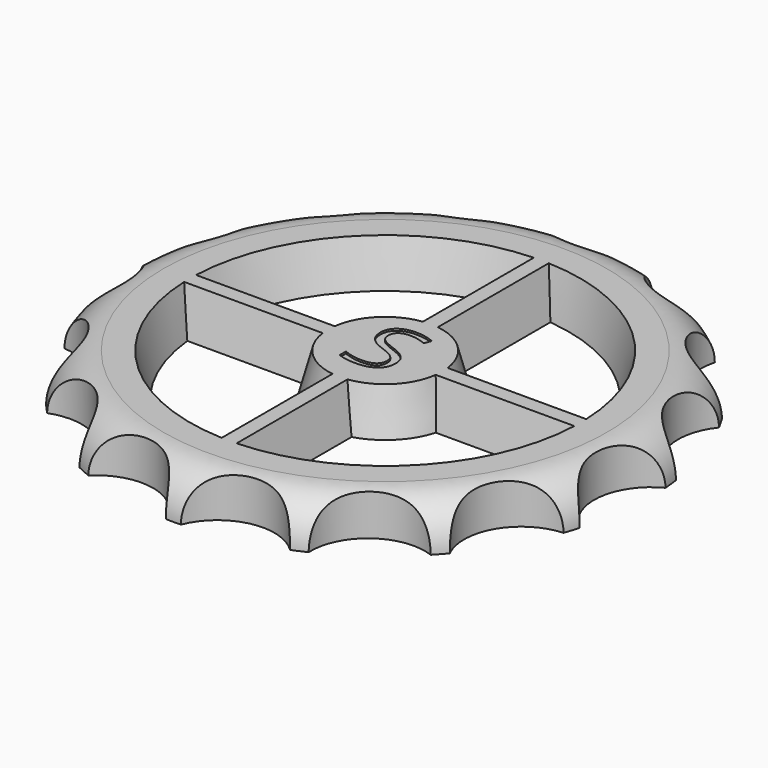
from build123d import *

# Parameters (mm, degrees)
F2_R                     = 15
F3_DEPTH                 = 25
F5_DEPTH                 = 25
DRAFT_F5_DRAFTED_ANGLE   = -15
DRAFT_F5_2_DRAFTED_ANGLE = -15
DRAFT_F5_3_DRAFTED_ANGLE = -15
DRAFT_F5_4_DRAFTED_ANGLE = -15
F6_TEXT_SIZE             = 25.1437097581
F7_DEPTH                 = 0.5


# Not quite as in the source:
# - an extrude with a draft is written as a straight extrude whose walls are then drafted
# - Text() gives the source's letters only with a copy of the font that has no kerning and outlines rounded to 1/6400 em; it was checked with that copy


with BuildPart() as f1:
    # F0 (on Front) → F1 (revolve)
    with BuildSketch(Plane.XZ):
        with BuildLine():
            Line((0, 11.3389009134), (-58.2126826048, 11.3389009134))
            ThreePointArc((-58.2126826048, 11.3389009134), (-66.2304963319, 8.0178137271), (-69.5515835182, 0))
            Line((-69.5515835182, 0), (0, 0))
            Line((0, 0), (0, 11.3389009134))
        make_face()
    revolve(axis=Axis((0, 0, 5.6694504567), (0, 0, 1)))

    # F2 (on Top) → F3 (cut)
    with BuildSketch(Plane.XY):
        with BuildLine():
            ThreePointArc((-0.9417421253, -75), (-12.820175043, -60.3284009409), (-29.6425179854, -68.8935492444))
            ThreePointArc((-29.6425179854, -68.8935492444), (-19.0633092075, -89.6715990591), (-0.9417421253, -75))
        make_face()
        with BuildLine():
            ThreePointArc((-30.0687543361, -62.0318186464), (-38.9650040167, -48.3298395179), (-55.1013186079, -50.8806907154))
            ThreePointArc((-55.1013186079, -50.8806907154), (-53.8855331205, -74.167073562), (-31.3631685962, -68.127466235))
            ThreePointArc((-31.3631685962, -68.127466235), (-30.3959259431, -65.1476021675), (-30.0687543361, -62.0318186464))
        make_face()
        with BuildLine():
            ThreePointArc((-51.4029694855, -38.3377723074), (-80.107353554, -32.2394235716), (-56.361617126, -49.4809874087))
            ThreePointArc((-56.361617126, -49.4809874087), (-52.698585417, -44.4361210433), (-51.4029694855, -38.3377723074))
        make_face()
        with BuildLine():
            Line((65.4227763465, 36.6844273957), (64.9519053636, 37.4999998618))
            ThreePointArc((64.9519053636, 37.4999998618), (65.1860656216, 37.0914659831), (65.4176563208, 36.6814700019))
            ThreePointArc((65.4176563208, 36.6814700019), (65.4202161879, 36.6829489511), (65.4227763465, 36.6844273957))
        make_face()
        with BuildLine():
            Line((44.8457793056, 60.1227324454), (44.0838958419, 60.6762731832))
            ThreePointArc((44.0838958419, 60.6762731832), (44.4639766809, 60.3983011162), (44.8423048098, 60.1179482297))
            ThreePointArc((44.8423048098, 60.1179482297), (44.844041822, 60.1203405087), (44.8457793056, 60.1227324454))
        make_face()
        with BuildLine():
            Line((44.0838958419, 60.6762731832), (43.3220085383, 61.2298167108))
            ThreePointArc((43.3220085383, 61.2298167108), (43.3202705833, 61.2274251166), (43.3185321569, 61.225033865))
            ThreePointArc((43.3185321569, 61.225033865), (43.7020753466, 60.9518548561), (44.0838958419, 60.6762731832))
        make_face()
        with BuildLine():
            ThreePointArc((43.3185321569, 61.225033865), (43.3202705833, 61.2274251166), (43.3220085383, 61.2298167108))
            ThreePointArc((43.3220085383, 61.2298167108), (45.4526013671, 65.4113405796), (46.1867536227, 70.0465954952))
            ThreePointArc((46.1867536227, 70.0465954952), (16.9218197284, 74.6846620097), (43.3185321569, 61.225033865))
        make_face()
        with BuildLine():
            ThreePointArc((71.9810342212, 51.305953661), (61.6162891368, 65.5718014055), (44.8457793056, 60.1227324454))
            ThreePointArc((44.8457793056, 60.1227324454), (44.844041822, 60.1203405087), (44.8423048098, 60.1179482297))
            ThreePointArc((44.8423048098, 60.1179482297), (45.833861839, 41.2689945657), (64.4759130302, 38.3126172289))
            ThreePointArc((64.4759130302, 38.3126172289), (64.4784737713, 38.3140946643), (64.4810342212, 38.3155726043))
            ThreePointArc((64.4810342212, 38.3155726043), (69.971415278, 43.805953661), (71.9810342212, 51.305953661))
        make_face()
        with BuildLine():
            ThreePointArc((64.4810342212, 38.3155726043), (64.4784737713, 38.3140946643), (64.4759130302, 38.3126172289))
            ThreePointArc((64.4759130302, 38.3126172289), (64.7151846964, 37.9070556719), (64.9519053636, 37.4999998618))
            Line((64.9519053636, 37.4999998618), (64.4810342212, 38.3155726043))
        make_face()
        with BuildLine():
            ThreePointArc((87.9227763465, 23.694046339), (80.4227763465, 36.6844273957), (65.4227763465, 36.6844273957))
            ThreePointArc((65.4227763465, 36.6844273957), (65.4202161879, 36.6829489511), (65.4176563208, 36.6814700019))
            ThreePointArc((65.4176563208, 36.6814700019), (65.4253367964, 10.7021873422), (87.9227763465, 23.694046339))
        make_face()
        with BuildLine():
            ThreePointArc((0, 61.6755446149), (10.6066017178, 66.0689428971), (15, 76.6755446149))
            ThreePointArc((15, 76.6755446149), (-10.6066017178, 87.2821463327), (0, 61.6755446149))
        make_face()
        with BuildLine():
            ThreePointArc((-16.5145396117, 73.1652708575), (-46.1045820532, 68.4786685462), (-16.1867536227, 70.0465954952))
            ThreePointArc((-16.1867536227, 70.0465954952), (-16.2689251921, 71.6145224442), (-16.5145396117, 73.1652708575))
        make_face()
        with Locations((-56.9810342212, 51.305953661)):
            Circle(F2_R)
        with Locations((-72.9227763465, 23.694046339)):
            Circle(F2_R)
        with Locations((-76.2555079588, -8.0147768488)):
            Circle(F2_R)
        with Locations((15.9417421253, -75)):
            Circle(F2_R)
        with Locations((45.0687543361, -62.0318186464)):
            Circle(F2_R)
        with Locations((66.4029694855, -38.3377723074)):
            Circle(F2_R)
        with Locations((76.2555079588, -8.0147768488)):
            Circle(F2_R)
    extrude(amount=F3_DEPTH, mode=Mode.SUBTRACT)


with BuildPart() as f5_drafted:
    # F4 (on face) → F5 (new body)
    with BuildSketch(Plane(origin=(0, 0, 0), x_dir=(1, 0, 0), z_dir=(0, 0, -1))):
        with BuildLine():
            Line((-5, 17.2916164658), (-5, 47.952713833))
            ThreePointArc((-5, 47.952713833), (-34.091514809, 34.091514809), (-47.952713833, 5))
            Line((-47.952713833, 5), (-17.2916164658, 5))
            ThreePointArc((-17.2916164658, 5), (-12.7279220614, 12.7279220614), (-5, 17.2916164658))
        make_face()
    extrude(amount=-F5_DEPTH)

    # draft_F5_drafted
    draft_f5_drafted_walls = [f5_drafted.faces().sort_by_distance(p)[0] for p in [
        (-32.6221651494, -5, 16.6666666667),
        (-12.7279220614, -12.7279220614, 16.6666666667),
        (-5, -32.6221651494, 16.6666666667),
        (-34.091514809, -34.091514809, 16.6666666667),
    ]]
    draft(draft_f5_drafted_walls, neutral_plane=Plane.XY, angle=DRAFT_F5_DRAFTED_ANGLE)


with BuildPart() as f1_1:
    add(f1.part)

    # join_F5_drafted: cut F5_drafted
    add(f5_drafted.part, mode=Mode.SUBTRACT)


with BuildPart() as f5_2_drafted:
    # F4 (on face) → F5, piece 2 (new body)
    with BuildSketch(Plane(origin=(0, 0, 0), x_dir=(1, 0, 0), z_dir=(0, 0, -1))):
        with BuildLine():
            Line((17.2916164658, 5), (47.952713833, 5))
            ThreePointArc((47.952713833, 5), (34.091514809, 34.091514809), (5, 47.952713833))
            Line((5, 47.952713833), (5, 17.2916164658))
            ThreePointArc((5, 17.2916164658), (12.7279220614, 12.7279220614), (17.2916164658, 5))
        make_face()
    extrude(amount=-F5_DEPTH)

    # draft_F5_2_drafted
    draft_f5_2_drafted_walls = [f5_2_drafted.faces().sort_by_distance(p)[0] for p in [
        (5, -32.6221651494, 16.6666666667),
        (12.7279220614, -12.7279220614, 16.6666666667),
        (32.6221651494, -5, 16.6666666667),
        (34.091514809, -34.091514809, 16.6666666667),
    ]]
    draft(draft_f5_2_drafted_walls, neutral_plane=Plane.XY, angle=DRAFT_F5_2_DRAFTED_ANGLE)


with BuildPart() as f1_2:
    add(f1_1.part)

    # join_F5_2_drafted: cut F5_2_drafted
    add(f5_2_drafted.part, mode=Mode.SUBTRACT)


with BuildPart() as f5_3_drafted:
    # F4 (on face) → F5, piece 3 (new body)
    with BuildSketch(Plane(origin=(0, 0, 0), x_dir=(1, 0, 0), z_dir=(0, 0, -1))):
        with BuildLine():
            ThreePointArc((5, -47.952713833), (34.091514809, -34.091514809), (47.952713833, -5))
            Line((47.952713833, -5), (17.2916164658, -5))
            ThreePointArc((17.2916164658, -5), (12.7279220614, -12.7279220614), (5, -17.2916164658))
            Line((5, -17.2916164658), (5, -47.952713833))
        make_face()
    extrude(amount=-F5_DEPTH)

    # draft_F5_3_drafted
    draft_f5_3_drafted_walls = [f5_3_drafted.faces().sort_by_distance(p)[0] for p in [
        (32.6221651494, 5, 16.6666666667),
        (12.7279220614, 12.7279220614, 16.6666666667),
        (5, 32.6221651494, 16.6666666667),
        (34.091514809, 34.091514809, 16.6666666667),
    ]]
    draft(draft_f5_3_drafted_walls, neutral_plane=Plane.XY, angle=DRAFT_F5_3_DRAFTED_ANGLE)


with BuildPart() as f1_3:
    add(f1_2.part)

    # join_F5_3_drafted: cut F5_3_drafted
    add(f5_3_drafted.part, mode=Mode.SUBTRACT)


with BuildPart() as f5_4_drafted:
    # F4 (on face) → F5, piece 4 (new body)
    with BuildSketch(Plane(origin=(0, 0, 0), x_dir=(1, 0, 0), z_dir=(0, 0, -1))):
        with BuildLine():
            ThreePointArc((-47.952713833, -5), (-34.091514809, -34.091514809), (-5, -47.952713833))
            Line((-5, -47.952713833), (-5, -17.2916164658))
            ThreePointArc((-5, -17.2916164658), (-12.7279220614, -12.7279220614), (-17.2916164658, -5))
            Line((-17.2916164658, -5), (-47.952713833, -5))
        make_face()
    extrude(amount=-F5_DEPTH)

    # draft_F5_4_drafted
    draft_f5_4_drafted_walls = [f5_4_drafted.faces().sort_by_distance(p)[0] for p in [
        (-5, 32.6221651494, 16.6666666667),
        (-12.7279220614, 12.7279220614, 16.6666666667),
        (-32.6221651494, 5, 16.6666666667),
        (-34.091514809, 34.091514809, 16.6666666667),
    ]]
    draft(draft_f5_4_drafted_walls, neutral_plane=Plane.XY, angle=DRAFT_F5_4_DRAFTED_ANGLE)


with BuildPart() as f1_4:
    add(f1_3.part)

    # join_F5_4_drafted: cut F5_4_drafted
    add(f5_4_drafted.part, mode=Mode.SUBTRACT)

    # F6 (on face) → F7 (cut)
    with BuildSketch(Plane.XY.offset(11.3389009134)):
        with Locations((-7.3227905668, -7.9439580441)):
            Text('S', F6_TEXT_SIZE, font='Open Sans', text_align=(TextAlign.LEFT, TextAlign.BOTTOM))
    extrude(amount=-F7_DEPTH, mode=Mode.SUBTRACT)


solid = f1_4.part
